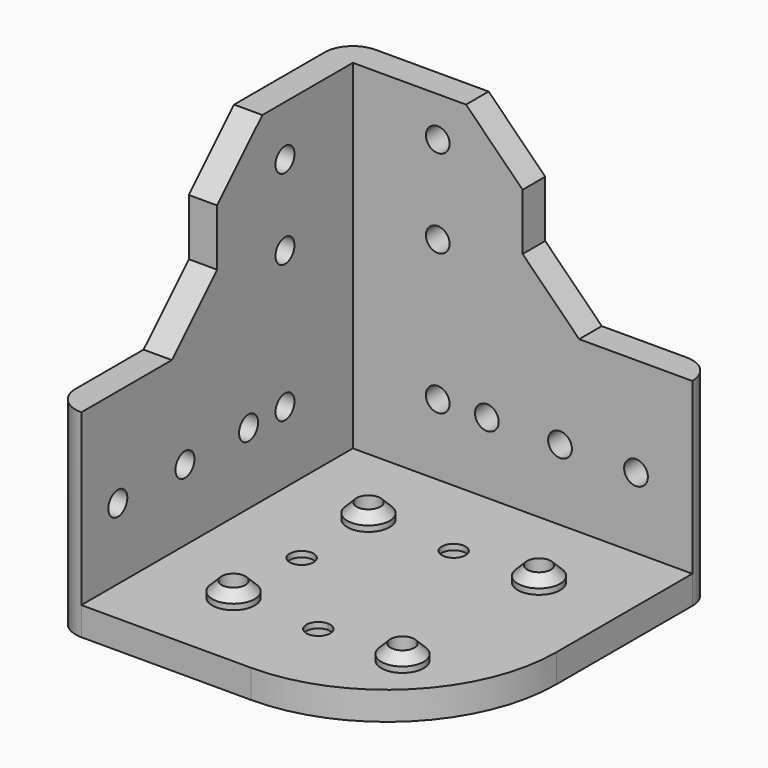
from build123d import *

# Parameters (mm, degrees)
F0_W      = 30
F0_H      = 30
F0_W_2    = 5
F0_H_2    = 5
F1_DEPTH  = 5
F2_DEPTH  = 35
F3_DEPTH  = 65
F4_R      = 2.1
F6_DEPTH  = 25
F5_R      = 2.1
F7_DEPTH  = 25
F8_R      = 3.75
F8_R_2    = 2.1
F9_DEPTH  = 4
F10_DEPTH = 25
F11_START = 4
F11_DEPTH = 4
F13_SIZE  = 10


# Not quite as in the source:
# - a fillet or chamfer that OpenCascade refuses, or shapes differently, is made with other operations: its cross-section is extruded or revolved along the edge and cut away or added


with BuildPart() as f1:
    # F0 (on Top) → F1 (new body)
    with BuildSketch(Plane.XY):
        with BuildLine():
            Line((-35, 30), (-30, 30))
            Line((-30, 30), (-30, 35))
            ThreePointArc((-30, 35), (-33.5355339059, 33.5355339059), (-35, 30))
        make_face()
        with Locations((15, 15)):
            Rectangle(F0_W, F0_H)
        with BuildLine():
            Line((0, 35), (0, 30))
            Line((0, 30), (30, 30))
            ThreePointArc((30, 30), (28.5355339059, 33.5355339059), (25, 35))
            Line((25, 35), (0, 35))
        make_face()
        with Locations((-15, -15)):
            Rectangle(F0_W, F0_H)
        with Locations((-32.5, 15)):
            Rectangle(F0_W_2, F0_H)
        with BuildLine():
            Line((30, 0), (0, 0))
            Line((0, 0), (0, -30))
            ThreePointArc((0, -30), (21.2132034356, -21.2132034356), (30, 0))
        make_face()
        with Locations((-15, 32.5)):
            Rectangle(F0_W, F0_H_2)
        with BuildLine():
            Line((-30, -30), (-30, 0))
            Line((-30, 0), (-35, 0))
            Line((-35, 0), (-35, -25))
            ThreePointArc((-35, -25), (-33.5355339059, -28.5355339059), (-30, -30))
        make_face()
        with Locations((-15, 15)):
            Rectangle(F0_W, F0_H)
    extrude(amount=F1_DEPTH)

    # F0 (on Top) → F2 (join)
    with BuildSketch(Plane.XY):
        with BuildLine():
            Line((-30, -30), (-30, 0))
            Line((-30, 0), (-35, 0))
            Line((-35, 0), (-35, -25))
            ThreePointArc((-35, -25), (-33.5355339059, -28.5355339059), (-30, -30))
        make_face()
        with Locations((-32.5, 15)):
            Rectangle(F0_W_2, F0_H)
        with BuildLine():
            Line((-35, 30), (-30, 30))
            Line((-30, 30), (-30, 35))
            ThreePointArc((-30, 35), (-33.5355339059, 33.5355339059), (-35, 30))
        make_face()
        with BuildLine():
            Line((0, 35), (0, 30))
            Line((0, 30), (30, 30))
            ThreePointArc((30, 30), (28.5355339059, 33.5355339059), (25, 35))
            Line((25, 35), (0, 35))
        make_face()
        with Locations((-15, 32.5)):
            Rectangle(F0_W, F0_H_2)
    extrude(amount=F2_DEPTH)

    # F0 (on Top) → F3 (join)
    with BuildSketch(Plane.XY):
        with Locations((-15, 32.5)):
            Rectangle(F0_W, F0_H_2)
        with BuildLine():
            Line((-35, 30), (-30, 30))
            Line((-30, 30), (-30, 35))
            ThreePointArc((-30, 35), (-33.5355339059, 33.5355339059), (-35, 30))
        make_face()
        with Locations((-32.5, 15)):
            Rectangle(F0_W_2, F0_H)
    extrude(amount=F3_DEPTH)

    # F4 (on face) → F6 (cut)
    with BuildSketch(Plane(origin=(0, 35, 0), x_dir=(-1, 0, 0), z_dir=(0, 1, 0))):
        with Locations((15, 17.5)):
            Circle(F4_R)
        with Locations((6.3242963515, 17.5)):
            Circle(F4_R)
        with Locations((-6.6132452339, 17.5)):
            Circle(F4_R)
        with Locations((-20.042758435, 17.5)):
            Circle(F4_R)
        with Locations((15, 42.3774681985)):
            Circle(F4_R)
        with Locations((15, 57.9239465296)):
            Circle(F4_R)
    extrude(amount=-F6_DEPTH, mode=Mode.SUBTRACT)

    # F5 (on face) → F7 (cut)
    with BuildSketch(Plane(origin=(-35, 0, 0), x_dir=(0, -1, 0), z_dir=(-1, 0, 0))):
        with Locations((21.9386201352, 17.5704155117)):
            Circle(F5_R)
        with Locations((7.1015073918, 17.5704155117)):
            Circle(F5_R)
        with Locations((-15, 17.5704155117)):
            Circle(F5_R)
        with Locations((-6.9537893869, 17.5704155117)):
            Circle(F5_R)
        with Locations((-15, 41.8734140694)):
            Circle(F5_R)
        with Locations((-15, 56.0644082725)):
            Circle(F5_R)
    extrude(amount=-F7_DEPTH, mode=Mode.SUBTRACT)

    # F8 (on face) → F9 (cut)
    with BuildSketch(Plane.XY):
        with Locations((-15.0563415678, 14.7660031606)):
            Circle(F8_R)
        with Locations((-15.0563415678, 14.7660031606)):
            Circle(F8_R_2, mode=Mode.SUBTRACT)
        with Locations((0, 14.7660031606)):
            Circle(F8_R)
        with Locations((0, 14.7660031606)):
            Circle(F8_R_2, mode=Mode.SUBTRACT)
        with Locations((15.0742138934, 14.7859862541)):
            Circle(F8_R)
        with Locations((15.0742138934, 14.7859862541)):
            Circle(F8_R_2, mode=Mode.SUBTRACT)
        with Locations((14.9396037335, -15.2109106032)):
            Circle(F8_R)
        with Locations((14.9396037335, -15.2109106032)):
            Circle(F8_R_2, mode=Mode.SUBTRACT)
        with Locations((0, -15.1403872296)):
            Circle(F8_R)
        with Locations((0, -15.1403872296)):
            Circle(F8_R_2, mode=Mode.SUBTRACT)
        with Locations((-14.9904824793, -15.1403872296)):
            Circle(F8_R)
        with Locations((-14.9904824793, -15.1403872296)):
            Circle(F8_R_2, mode=Mode.SUBTRACT)
        with Locations((-15.0563415678, 0)):
            Circle(F8_R)
        with Locations((-15.0563415678, 0)):
            Circle(F8_R_2, mode=Mode.SUBTRACT)
    extrude(amount=F9_DEPTH, mode=Mode.SUBTRACT)

    # F8 (on face) → F10 (cut)
    with BuildSketch(Plane.XY):
        with Locations((-14.9904824793, -15.1403872296)):
            Circle(F8_R_2)
        with BuildLine():
            Line((0, -17.2403872296), (0, -13.0403872296))
            ThreePointArc((0, -13.0403872296), (-2.1, -15.1403872296), (0, -17.2403872296))
        make_face()
        with BuildLine():
            ThreePointArc((2.1, -15.1403872296), (1.4849242405, -13.6554629891), (0, -13.0403872296))
            Line((0, -13.0403872296), (0, -17.2403872296))
            ThreePointArc((0, -17.2403872296), (1.4849242405, -16.6253114701), (2.1, -15.1403872296))
        make_face()
        with Locations((14.9396037335, -15.2109106032)):
            Circle(F8_R_2)
        with Locations((15.0742138934, 14.7859862541)):
            Circle(F8_R_2)
        with Locations((0, 14.7660031606)):
            Circle(F8_R_2)
        with Locations((-15.0563415678, 14.7660031606)):
            Circle(F8_R_2)
        with BuildLine():
            Line((-17.1563415678, 0), (-12.9563415678, 0))
            ThreePointArc((-12.9563415678, 0), (-15.0563415678, 2.1), (-17.1563415678, 0))
        make_face()
        with BuildLine():
            ThreePointArc((-17.1563415678, 0), (-15.0563415678, -2.1), (-12.9563415678, 0))
            Line((-12.9563415678, 0), (-17.1563415678, 0))
        make_face()
    extrude(amount=F10_DEPTH, mode=Mode.SUBTRACT)

    # F8 (on face) → F11 (join)
    with BuildSketch(Plane.XY.offset(F11_START)):
        with Locations((-14.9904824793, -15.1403872296)):
            Circle(F8_R)
        with Locations((-14.9904824793, -15.1403872296)):
            Circle(F8_R_2, mode=Mode.SUBTRACT)
        with Locations((14.9396037335, -15.2109106032)):
            Circle(F8_R)
        with Locations((14.9396037335, -15.2109106032)):
            Circle(F8_R_2, mode=Mode.SUBTRACT)
        with Locations((-15.0563415678, 14.7660031606)):
            Circle(F8_R)
        with Locations((-15.0563415678, 14.7660031606)):
            Circle(F8_R_2, mode=Mode.SUBTRACT)
        with Locations((15.0742138934, 14.7859862541)):
            Circle(F8_R)
        with Locations((15.0742138934, 14.7859862541)):
            Circle(F8_R_2, mode=Mode.SUBTRACT)
    extrude(amount=F11_DEPTH)

    # F12: chamfer of 2 on 4 edges, made by hand

    # F12_s1 → F12_t2 (revolve, cut)
    with BuildSketch(Plane.XZ.offset(-14.7660031606)):
        Polygon((-11.3063415678, 6), (-13.3063415678, 8), (-11.3063415678, 8), align=None)
    revolve(axis=Axis((-15.0563415678, 14.7660031606, 8), (0, 0, 1)), mode=Mode.SUBTRACT)

    # F12_s3 → F12_t4 (revolve, cut)
    with BuildSketch(Plane.XZ.offset(-14.7859862541)):
        Polygon((18.8242138934, 6), (16.8242138934, 8), (18.8242138934, 8), align=None)
    revolve(axis=Axis((15.0742138934, 14.7859862541, 8), (0, 0, 1)), mode=Mode.SUBTRACT)

    # F12_s5 → F12_t6 (revolve, cut)
    with BuildSketch(Plane.XZ.offset(15.2109106032)):
        Polygon((18.6896037335, 6), (16.6896037335, 8), (18.6896037335, 8), align=None)
    revolve(axis=Axis((14.9396037335, -15.2109106032, 8), (0, 0, 1)), mode=Mode.SUBTRACT)

    # F12_s7 → F12_t8 (revolve, cut)
    with BuildSketch(Plane.XZ.offset(15.1403872296)):
        Polygon((-11.2404824793, 6), (-13.2404824793, 8), (-11.2404824793, 8), align=None)
    revolve(axis=Axis((-14.9904824793, -15.1403872296, 8), (0, 0, 1)), mode=Mode.SUBTRACT)

    # F13
    f13_edges = [f1.edges().sort_by_distance(p)[0] for p in [
        (-32.5, 0, 65),
        (0, 32.5, 65),
        (-32.5, 0, 35),
        (0, 32.5, 35),
    ]]
    chamfer(f13_edges, length=F13_SIZE)


solid = f1.part
